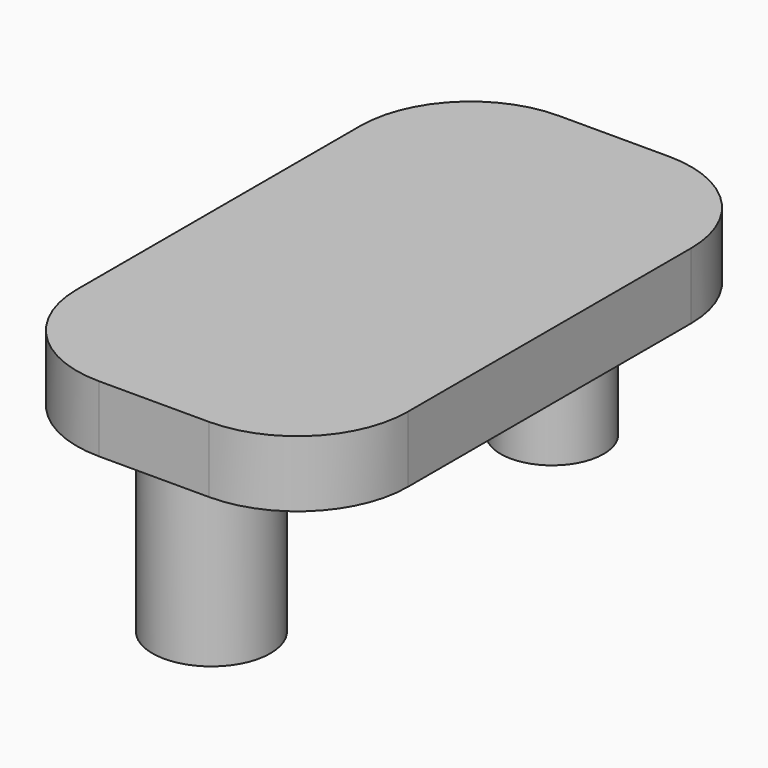
from build123d import *

# Parameters (mm, degrees)
F0_R     = 2.675
F1_DEPTH = 7.5
F0_R_2   = 2.3375
F2_W     = 15
F2_H     = 7
F2_R     = 2.3375
F2_H_2   = 12.555
F2_H_3   = 6.5
F3_DEPTH = 3
F4_R     = 5


# Not quite as in the source:
# - a feature names something its author has since deleted; it is built from what else it names


with BuildPart() as f1:
    # F0 (on Top) → F1 (new body)
    with BuildSketch(Plane.XY):
        Circle(F0_R)
    extrude(amount=F1_DEPTH)



with BuildPart() as f1b:
    # F0 (on Top) → F1, piece 2 (new body)
    with BuildSketch(Plane.XY):
        with Locations((0, 19.305)):
            Circle(F0_R_2)
    extrude(amount=F1_DEPTH)


with BuildPart() as f1_1:
    add(f1.part)

    add(f1b.part)  # F3 merges F1b
    # F2 (on face) → F3 (join)
    with BuildSketch(Plane.XY.offset(7.5)):
        with Locations((0, 19.305)):
            Rectangle(F2_W, F2_H)
        with Locations((0, 19.305)):
            Circle(F2_R, mode=Mode.SUBTRACT)
        with Locations((0, 19.305)):
            Circle(F2_R)
        with Locations((0, 9.5275)):
            Rectangle(F2_W, F2_H_2)
        Rectangle(F2_W, F2_H_3)
    extrude(amount=F3_DEPTH)

    # F4
    f4_edges = [f1_1.edges().sort_by_distance(p)[0] for p in [
        (-7.5, -3.25, 9),
        (7.5, -3.25, 9),
        (7.5, 22.805, 9),
        (-7.5, 22.805, 9),
    ]]
    fillet(f4_edges, radius=F4_R)


solid = f1_1.part
